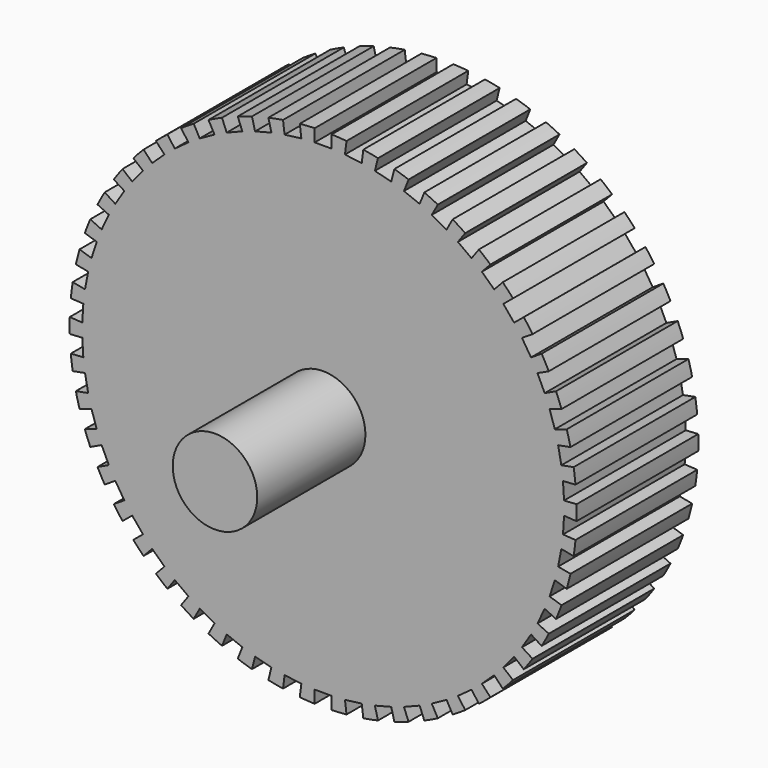
from build123d import *

# Parameters (mm, degrees)
F0_R            = 30
F0_R_2          = 5
F1_DEPTH        = 9
F2_DEPTH        = 25
F3_W            = 2
F3_H            = 3
F4_DEPTH        = 34.001
F4_COPIES_COUNT = 50


# Not quite as in the source:
# - a pattern or mirror of a feature is missing from the dataset's text; its kind, count and spacing are read off the source's solid


with BuildPart() as f1:
    # F0 (on Front) → F1 (new body, symmetric)
    with BuildSketch(Plane.XZ):
        Circle(F0_R)
        Circle(F0_R_2, mode=Mode.SUBTRACT)
    extrude(amount=F1_DEPTH, both=True)

    # F0 (on Front) → F2 (join, symmetric)
    with BuildSketch(Plane.XZ):
        Circle(F0_R_2)
    extrude(amount=F2_DEPTH, both=True)

    # F3 (on face) → F4 (cut, through all)
    with BuildSketch(Plane.XZ.offset(9)):
        with Locations((0, 30)):
            Rectangle(F3_W, F3_H)
    f4 = extrude(amount=-F4_DEPTH, mode=Mode.SUBTRACT)

    # F4_copies: F4 ×50 about axis
    f4_copies_axis = Axis((0, 0, 0), (0, 1, 0))
    for i in range(1, F4_COPIES_COUNT):
        add(f4.rotate(f4_copies_axis, i * 360 / F4_COPIES_COUNT), mode=Mode.SUBTRACT)


solid = f1.part
